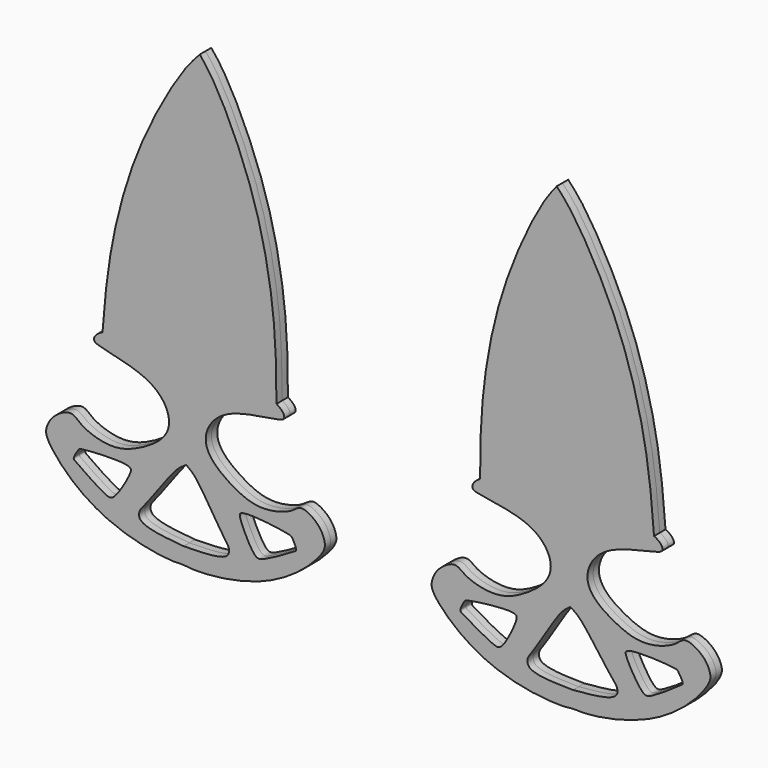
from build123d import *

# Parameters (mm, degrees)
F1_DEPTH = 2.62151


with BuildPart() as f1:
    # F0 (on Front) → F1 (new body, symmetric)
    with BuildSketch(Plane.XZ):
        with BuildLine():
            add(Edge.make_bspline(
                [(-42.2445336557, -130.09934769), (-43.750003111, -130.1677806227), (-47.5235789543, -130.3393130711), (-59.0286199188, -128.4700613421), (-72.1811760889, -123.9628181948), (-84.7164617577, -115.3912526778), (-92.6003041855, -105.4851726011), (-92.1103858513, -101.8336882182), (-89.9748357868, -97.4877733415), (-82.8389972388, -93.4017797473), (-79.6123226782, -97.8246997119), (-68.3837596427, -101.661771716), (-57.7999215333, -98.1865176664), (-44.145076362, -89.1421245094), (-51.5740810802, -72.7966063898), (-73.4787077419, -70.4160463532), (-75.2301228368, -67.9896103093), (-73.7265465215, -65.939554609), (-71.6269252491, -64.9718962005)],
                knots=[0, 0, 0, 0, 0.0332821358, 0.0834242523, 0.1394389336, 0.1985912257, 0.2494938822, 0.275648302, 0.3081433735, 0.3472533821, 0.3788314128, 0.4280288211, 0.4786379304, 0.5336428238, 0.5889527046, 0.6566534811, 0.6765070934, 0.7076101155, 0.7076101155, 0.7076101155, 0.7076101155], degree=3))
            add(Edge.make_bspline(
                [(-42.2445336557, -130.09934769), (-40.7482509334, -130.2789566039), (-36.9977023481, -130.7291602637), (-25.3859086453, -129.7160874006), (-11.9359744285, -126.1941214498), (1.1990288738, -118.5733071587), (9.7940501024, -109.2775552261), (9.5755837516, -105.5998343793), (7.767363068, -101.1078539528), (0.9533262657, -96.5051984267), (-2.5916829216, -100.6773153469), (-14.0733209231, -103.6732689864), (-24.3710887004, -99.424622303), (-37.3194862046, -89.3949240871), (-28.701714672, -73.6437308779), (-6.6810044769, -72.8900347974), (-4.7548980287, -70.5998032238), (-6.1027070374, -68.4441406839), (-8.1249957307, -67.3238189782)],
                knots=[0, 0, 0, 0, 0.0332821358, 0.0834242523, 0.1394389336, 0.1985912257, 0.2494938822, 0.275648302, 0.3081433735, 0.3472533821, 0.3788314128, 0.4280288211, 0.4786379304, 0.5336428238, 0.5889527046, 0.6566534811, 0.6765070934, 0.7076101155, 0.7076101155, 0.7076101155, 0.7076101155], degree=3))
            add(Edge.make_bspline(
                [(-8.1249957307, -67.3238189782), (-12.0171270025, -65.167628737), (-26.1680261667, -62.7362957146), (-22.7153994707, -52.0755739194), (-25.9462625771, -3.5065694424), (-36.2441394619, 22.9051794418), (-36.5819767147, 22.7897246783)],
                knots=[0.7076101155, 0.7076101155, 0.7076101155, 0.7076101155, 0.7674715217, 0.8092327738, 0.9176213096, 0.9912848605, 0.9912848605, 0.9912848605, 0.9912848605], degree=3))
            add(Edge.make_bspline(
                [(-71.6269252491, -64.9718962005), (-67.585958378, -63.1095243419), (-53.293976792, -61.7316311064), (-55.9485430827, -50.8447170301), (-49.1337567977, -2.6477735565), (-36.9103478989, 22.9298538227), (-36.5819767147, 22.7897246783)],
                knots=[0.7076101155, 0.7076101155, 0.7076101155, 0.7076101155, 0.7674715217, 0.8092327738, 0.9176213096, 0.9912848605, 0.9912848605, 0.9912848605, 0.9912848605], degree=3))
        make_face()
        with BuildLine():
            add(Edge.make_bspline(
                [(-79.2514724494, -105.0157840501), (-80.0857124514, -105.1576394879), (-80.3591992691, -105.4704049062), (-82.554508259, -108.8750564811), (-81.2578172887, -109.8483305625), (-70.6015356744, -117.2850725962), (-67.158405392, -117.4279735341), (-61.2406938044, -107.3490957269), (-60.8877661151, -103.590157875), (-76.3891136813, -104.5290642152), (-79.2514724494, -105.0157840501)],
                knots=[0, 0, 0, 0, 0.0652750561, 0.1639305927, 0.2265744696, 0.4193396501, 0.5157256644, 0.6954966114, 0.7760349196, 1, 1, 1, 1], degree=3))
        make_face(mode=Mode.SUBTRACT)
        with BuildLine():
            add(Edge.make_bspline(
                [(-41.0430528272, -97.6593579035), (-42.061383527, -98.2770837815), (-44.6857579552, -99.8690459982), (-50.1102026655, -107.4261895027), (-56.6058960283, -116.0795918607), (-58.2671680567, -117.8286447153), (-58.7175678133, -122.563739407), (-48.9449955926, -123.4442438978), (-42.0211533871, -124.0680790579)],
                knots=[0, 0, 0, 0, 0.1270993549, 0.3275520388, 0.5387517331, 0.6366858314, 0.7425928489, 1, 1, 1, 1], degree=3))
            add(Edge.make_bspline(
                [(-41.0430528272, -97.6593579035), (-40.0732068539, -98.3507199378), (-37.5737840511, -100.1324523789), (-32.7232222732, -108.0701515922), (-26.8854398715, -117.1803492444), (-25.3581012337, -119.0474987634), (-25.2592026472, -123.8029378335), (-35.0701339036, -123.9581275466), (-42.0211533871, -124.0680790579)],
                knots=[0, 0, 0, 0, 0.1270993549, 0.3275520388, 0.5387517331, 0.6366858314, 0.7425928489, 1, 1, 1, 1], degree=3))
        make_face(mode=Mode.SUBTRACT)
        with BuildLine():
            add(Edge.make_bspline(
                [(-3.4834876238, -107.8220050687), (-2.6620266234, -108.0251827518), (-2.412425151, -108.357321806), (-0.4749815846, -111.9150382554), (-1.8401155791, -112.7897262495), (-13.0173169533, -119.41782095), (-16.4615847582, -119.3056331283), (-21.6175227908, -108.8166202437), (-21.6914252023, -105.0418738731), (-6.3020003919, -107.1248826323), (-3.4834876238, -107.8220050687)],
                knots=[0, 0, 0, 0, 0.0652750561, 0.1639305927, 0.2265744696, 0.4193396501, 0.5157256644, 0.6954966114, 0.7760349196, 1, 1, 1, 1], degree=3))
        make_face(mode=Mode.SUBTRACT)
        with BuildLine():
            add(Edge.make_bspline(
                [(-36.5819767147, 22.7897246783), (-36.621946262, 22.7760652177), (-36.6083205058, 22.6112014371), (-36.5946947496, 22.4463376565)],
                knots=[0.9912848605, 0.9912848605, 0.9912848605, 0.9912848605, 1, 1, 1, 1], degree=3))
            add(Edge.make_bspline(
                [(-36.5819767147, 22.7897246783), (-36.5431270985, 22.7731459901), (-36.568910924, 22.6097418233), (-36.5946947496, 22.4463376565)],
                knots=[0.9912848605, 0.9912848605, 0.9912848605, 0.9912848605, 1, 1, 1, 1], degree=3))
        make_face(mode=Mode.SUBTRACT)
        with BuildLine():
            add(Edge.make_bspline(
                [(-71.6269252491, -64.9718962005), (-70.9757488216, -56.7243907236), (-69.5310005896, -38.4258644656), (-60.483849714, -2.374428068), (-43.2893475448, 28.1428030298), (-37.9466087075, 33.8959019702), (-36.0968659606, 35.8877180334)],
                knots=[0, 0, 0, 0, 0.2514200282, 0.5578190884, 0.8469098043, 1, 1, 1, 1], degree=3))
            add(Edge.make_bspline(
                [(-71.6269252491, -64.9718962005), (-67.585958378, -63.1095243419), (-53.293976792, -61.7316311064), (-55.9485430827, -50.8447170301), (-49.1337567977, -2.6477735565), (-36.9103478989, 22.9298538227), (-36.5819767147, 22.7897246783)],
                knots=[0.7076101155, 0.7076101155, 0.7076101155, 0.7076101155, 0.7674715217, 0.8092327738, 0.9176213096, 0.9912848605, 0.9912848605, 0.9912848605, 0.9912848605], degree=3))
            add(Edge.make_bspline(
                [(-8.1249957307, -67.3238189782), (-12.0171270025, -65.167628737), (-26.1680261667, -62.7362957146), (-22.7153994707, -52.0755739194), (-25.9462625771, -3.5065694424), (-36.2441394619, 22.9051794418), (-36.5819767147, 22.7897246783)],
                knots=[0.7076101155, 0.7076101155, 0.7076101155, 0.7076101155, 0.7674715217, 0.8092327738, 0.9176213096, 0.9912848605, 0.9912848605, 0.9912848605, 0.9912848605], degree=3))
            add(Edge.make_bspline(
                [(-8.1249957307, -67.3238189782), (-8.1642988068, -59.0507401922), (-8.2514995214, -40.6954750973), (-14.6070457189, -4.0735685681), (-29.4970011866, 27.6319755037), (-34.3995307845, 33.7645287438), (-36.0968659606, 35.8877180334)],
                knots=[0, 0, 0, 0, 0.2514200282, 0.5578190884, 0.8469098043, 1, 1, 1, 1], degree=3))
        make_face()
    extrude(amount=F1_DEPTH, both=True)


with BuildPart() as f1b:
    # F0 (on Front) → F1, piece 2 (new body, symmetric)
    with BuildSketch(Plane.XZ):
        with BuildLine():
            add(Edge.make_bspline(
                [(66.2170385344, -67.3238189782), (70.1091698063, -65.167628737), (84.2600689705, -62.7362957146), (80.8074422745, -52.0755739194), (84.0383053808, -3.5065694424), (94.3361822657, 22.9051794418), (94.6740195184, 22.7897246783)],
                knots=[0.7076101155, 0.7076101155, 0.7076101155, 0.7076101155, 0.7674715217, 0.8092327738, 0.9176213096, 0.9912848605, 0.9912848605, 0.9912848605, 0.9912848605], degree=3))
            add(Edge.make_bspline(
                [(100.3365764595, -130.09934769), (98.8402937371, -130.2789566039), (95.0897451519, -130.7291602637), (83.4779514491, -129.7160874006), (70.0280172322, -126.1941214498), (56.8930139299, -118.5733071587), (48.2979927014, -109.2775552261), (48.5164590522, -105.5998343793), (50.3246797358, -101.1078539528), (57.1387165381, -96.5051984267), (60.6837257253, -100.6773153469), (72.1653637269, -103.6732689864), (82.4631315041, -99.424622303), (95.4115290084, -89.3949240871), (86.7937574758, -73.6437308779), (64.7730472807, -72.8900347974), (62.8469408324, -70.5998032238), (64.1947498412, -68.4441406839), (66.2170385344, -67.3238189782)],
                knots=[0, 0, 0, 0, 0.0332821358, 0.0834242523, 0.1394389336, 0.1985912257, 0.2494938822, 0.275648302, 0.3081433735, 0.3472533821, 0.3788314128, 0.4280288211, 0.4786379304, 0.5336428238, 0.5889527046, 0.6566534811, 0.6765070934, 0.7076101155, 0.7076101155, 0.7076101155, 0.7076101155], degree=3))
            add(Edge.make_bspline(
                [(100.3365764595, -130.09934769), (101.8420459148, -130.1677806227), (105.6156217581, -130.3393130711), (117.1206627226, -128.4700613421), (130.2732188927, -123.9628181948), (142.8085045614, -115.3912526778), (150.6923469893, -105.4851726011), (150.202428655, -101.8336882182), (148.0668785906, -97.4877733415), (140.9310400426, -93.4017797473), (137.704365482, -97.8246997119), (126.4758024464, -101.661771716), (115.8919643371, -98.1865176664), (102.2371191657, -89.1421245094), (109.6661238839, -72.7966063898), (131.5707505456, -70.4160463532), (133.3221656406, -67.9896103093), (131.8185893253, -65.939554609), (129.7189680529, -64.9718962005)],
                knots=[0, 0, 0, 0, 0.0332821358, 0.0834242523, 0.1394389336, 0.1985912257, 0.2494938822, 0.275648302, 0.3081433735, 0.3472533821, 0.3788314128, 0.4280288211, 0.4786379304, 0.5336428238, 0.5889527046, 0.6566534811, 0.6765070934, 0.7076101155, 0.7076101155, 0.7076101155, 0.7076101155], degree=3))
            add(Edge.make_bspline(
                [(129.7189680529, -64.9718962005), (125.6780011817, -63.1095243419), (111.3860195958, -61.7316311064), (114.0405858864, -50.8447170301), (107.2257996014, -2.6477735565), (95.0023907027, 22.9298538227), (94.6740195184, 22.7897246783)],
                knots=[0.7076101155, 0.7076101155, 0.7076101155, 0.7076101155, 0.7674715217, 0.8092327738, 0.9176213096, 0.9912848605, 0.9912848605, 0.9912848605, 0.9912848605], degree=3))
        make_face()
        with BuildLine():
            add(Edge.make_bspline(
                [(61.5755304276, -107.8220050687), (60.7540694272, -108.0251827518), (60.5044679548, -108.357321806), (58.5670243883, -111.9150382554), (59.9321583829, -112.7897262495), (71.109359757, -119.41782095), (74.553627562, -119.3056331283), (79.7095655945, -108.8166202437), (79.783468006, -105.0418738731), (64.3940431957, -107.1248826323), (61.5755304276, -107.8220050687)],
                knots=[0, 0, 0, 0, 0.0652750561, 0.1639305927, 0.2265744696, 0.4193396501, 0.5157256644, 0.6954966114, 0.7760349196, 1, 1, 1, 1], degree=3))
        make_face(mode=Mode.SUBTRACT)
        with BuildLine():
            add(Edge.make_bspline(
                [(99.135095631, -97.6593579035), (98.1652496577, -98.3507199378), (95.6658268549, -100.1324523789), (90.8152650769, -108.0701515922), (84.9774826753, -117.1803492444), (83.4501440374, -119.0474987634), (83.3512454509, -123.8029378335), (93.1621767074, -123.9581275466), (100.1131961908, -124.0680790579)],
                knots=[0, 0, 0, 0, 0.1270993549, 0.3275520388, 0.5387517331, 0.6366858314, 0.7425928489, 1, 1, 1, 1], degree=3))
            add(Edge.make_bspline(
                [(99.135095631, -97.6593579035), (100.1534263308, -98.2770837815), (102.7778007589, -99.8690459982), (108.2022454693, -107.4261895027), (114.697938832, -116.0795918607), (116.3592108605, -117.8286447153), (116.809610617, -122.563739407), (107.0370383964, -123.4442438978), (100.1131961908, -124.0680790579)],
                knots=[0, 0, 0, 0, 0.1270993549, 0.3275520388, 0.5387517331, 0.6366858314, 0.7425928489, 1, 1, 1, 1], degree=3))
        make_face(mode=Mode.SUBTRACT)
        with BuildLine():
            add(Edge.make_bspline(
                [(137.3435152532, -105.0157840501), (138.1777552551, -105.1576394879), (138.4512420729, -105.4704049062), (140.6465510628, -108.8750564811), (139.3498600924, -109.8483305625), (128.6935784782, -117.2850725962), (125.2504481958, -117.4279735341), (119.3327366081, -107.3490957269), (118.9798089188, -103.590157875), (134.481156485, -104.5290642152), (137.3435152532, -105.0157840501)],
                knots=[0, 0, 0, 0, 0.0652750561, 0.1639305927, 0.2265744696, 0.4193396501, 0.5157256644, 0.6954966114, 0.7760349196, 1, 1, 1, 1], degree=3))
        make_face(mode=Mode.SUBTRACT)
        with BuildLine():
            add(Edge.make_bspline(
                [(94.6740195184, 22.7897246783), (94.6351699023, 22.7731459901), (94.6609537278, 22.6097418233), (94.6867375534, 22.4463376565)],
                knots=[0.9912848605, 0.9912848605, 0.9912848605, 0.9912848605, 1, 1, 1, 1], degree=3))
            add(Edge.make_bspline(
                [(94.6740195184, 22.7897246783), (94.7139890658, 22.7760652177), (94.7003633096, 22.6112014371), (94.6867375534, 22.4463376565)],
                knots=[0.9912848605, 0.9912848605, 0.9912848605, 0.9912848605, 1, 1, 1, 1], degree=3))
        make_face(mode=Mode.SUBTRACT)
        with BuildLine():
            add(Edge.make_bspline(
                [(66.2170385344, -67.3238189782), (66.2563416106, -59.0507401922), (66.3435423252, -40.6954750973), (72.6990885226, -4.0735685681), (87.5890439903, 27.6319755037), (92.4915735882, 33.7645287438), (94.1889087644, 35.8877180334)],
                knots=[0, 0, 0, 0, 0.2514200282, 0.5578190884, 0.8469098043, 1, 1, 1, 1], degree=3))
            add(Edge.make_bspline(
                [(66.2170385344, -67.3238189782), (70.1091698063, -65.167628737), (84.2600689705, -62.7362957146), (80.8074422745, -52.0755739194), (84.0383053808, -3.5065694424), (94.3361822657, 22.9051794418), (94.6740195184, 22.7897246783)],
                knots=[0.7076101155, 0.7076101155, 0.7076101155, 0.7076101155, 0.7674715217, 0.8092327738, 0.9176213096, 0.9912848605, 0.9912848605, 0.9912848605, 0.9912848605], degree=3))
            add(Edge.make_bspline(
                [(129.7189680529, -64.9718962005), (125.6780011817, -63.1095243419), (111.3860195958, -61.7316311064), (114.0405858864, -50.8447170301), (107.2257996014, -2.6477735565), (95.0023907027, 22.9298538227), (94.6740195184, 22.7897246783)],
                knots=[0.7076101155, 0.7076101155, 0.7076101155, 0.7076101155, 0.7674715217, 0.8092327738, 0.9176213096, 0.9912848605, 0.9912848605, 0.9912848605, 0.9912848605], degree=3))
            add(Edge.make_bspline(
                [(129.7189680529, -64.9718962005), (129.0677916254, -56.7243907236), (127.6230433933, -38.4258644656), (118.5758925178, -2.374428068), (101.3813903485, 28.1428030298), (96.0386515113, 33.8959019702), (94.1889087644, 35.8877180334)],
                knots=[0, 0, 0, 0, 0.2514200282, 0.5578190884, 0.8469098043, 1, 1, 1, 1], degree=3))
        make_face()
    extrude(amount=F1_DEPTH, both=True)


solid = Compound([f1.part, f1b.part])
